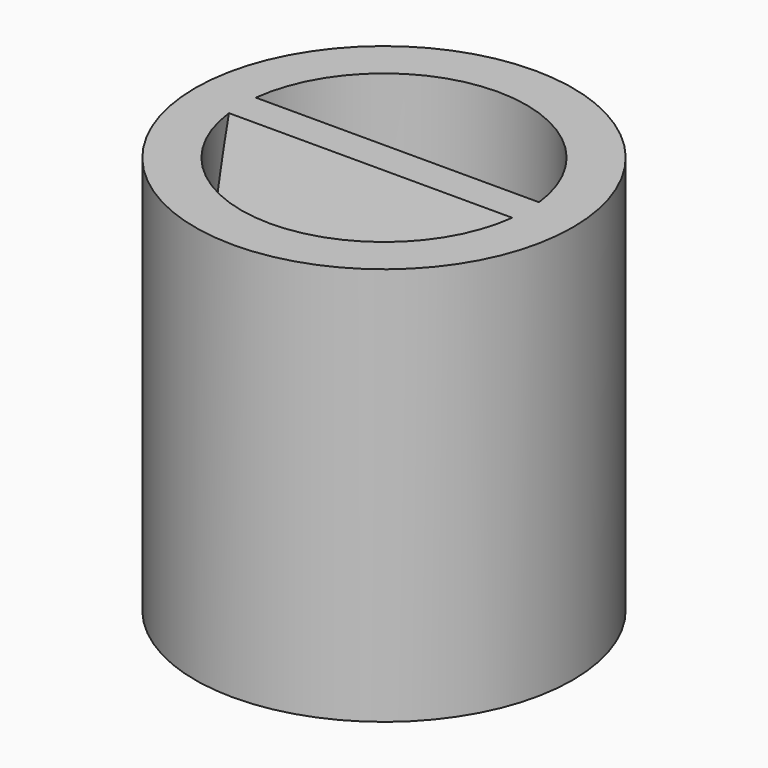
from build123d import *

# Parameters (mm, degrees)
F0_R       = 4.5
F1_DEPTH   = 8
F2_SIZE2   = 0.6
F2_SIZE    = 2
F2_2_SIZE2 = 0.6
F2_2_SIZE  = 2
F3_DEPTH   = 1.5


# Not quite as in the source:
# - a feature names something its author has since deleted; it is built from what else it names


with BuildPart() as f1:
    # F0 (on Top) → F1 (new body)
    with BuildSketch(Plane.XY):
        Circle(F0_R)
        with BuildLine():
            ThreePointArc((3.2496153619, 1), (3.3621936463, 0.5056222749), (3.4, 0))
            ThreePointArc((3.4, 0), (3.3621936463, -0.5056222749), (3.2496153619, -1))
            ThreePointArc((3.2496153619, -1), (0, -3.4), (-3.2496153619, -1))
            ThreePointArc((-3.2496153619, -1), (-3.4, 0), (-3.2496153619, 1))
            ThreePointArc((-3.2496153619, 1), (0, 3.4), (3.2496153619, 1))
        make_face(mode=Mode.SUBTRACT)
        with BuildLine():
            ThreePointArc((3.2496153619, -1), (3.3621936463, -0.5056222749), (3.4, 0))
            ThreePointArc((3.4, 0), (3.3621936463, 0.5056222749), (3.2496153619, 1))
            Line((3.2496153619, 1), (-3.2496153619, 1))
            ThreePointArc((-3.2496153619, 1), (-3.4, 0), (-3.2496153619, -1))
            Line((-3.2496153619, -1), (3.2496153619, -1))
        make_face()
    extrude(amount=F1_DEPTH)

    # F2
    f2_edges = [f1.edges().sort_by_distance(p)[0] for p in [
        (0, 1, 8),
    ]]
    f2_side = f1.faces().sort_by_distance((0, 1, 4))[0]
    chamfer(f2_edges, length=F2_SIZE, length2=F2_SIZE2, reference=f2_side)

    # F2#2
    f2_2_edges = [f1.edges().sort_by_distance(p)[0] for p in [
        (0, -1, 8),
    ]]
    f2_2_side = f1.faces().sort_by_distance((0, -1, 4))[0]
    chamfer(f2_2_edges, length=F2_2_SIZE, length2=F2_2_SIZE2, reference=f2_2_side)

    # F0 (on Top) → F3 (join)
    with BuildSketch(Plane.XY):
        Circle(F0_R)
        with BuildLine():
            ThreePointArc((3.2496153619, 1), (3.3621936463, 0.5056222749), (3.4, 0))
            ThreePointArc((3.4, 0), (3.3621936463, -0.5056222749), (3.2496153619, -1))
            ThreePointArc((3.2496153619, -1), (0, -3.4), (-3.2496153619, -1))
            ThreePointArc((-3.2496153619, -1), (-3.4, 0), (-3.2496153619, 1))
            ThreePointArc((-3.2496153619, 1), (0, 3.4), (3.2496153619, 1))
        make_face(mode=Mode.SUBTRACT)
        with BuildLine():
            ThreePointArc((3.2496153619, -1), (3.3621936463, -0.5056222749), (3.4, 0))
            ThreePointArc((3.4, 0), (3.3621936463, 0.5056222749), (3.2496153619, 1))
            Line((3.2496153619, 1), (-3.2496153619, 1))
            ThreePointArc((-3.2496153619, 1), (-3.4, 0), (-3.2496153619, -1))
            Line((-3.2496153619, -1), (3.2496153619, -1))
        make_face()
        with BuildLine():
            Line((-3.2496153619, 1), (3.2496153619, 1))
            ThreePointArc((3.2496153619, 1), (0, 3.4), (-3.2496153619, 1))
        make_face()
        with BuildLine():
            ThreePointArc((-3.2496153619, -1), (0, -3.4), (3.2496153619, -1))
            Line((3.2496153619, -1), (-3.2496153619, -1))
        make_face()
    extrude(amount=-F3_DEPTH)


solid = f1.part
